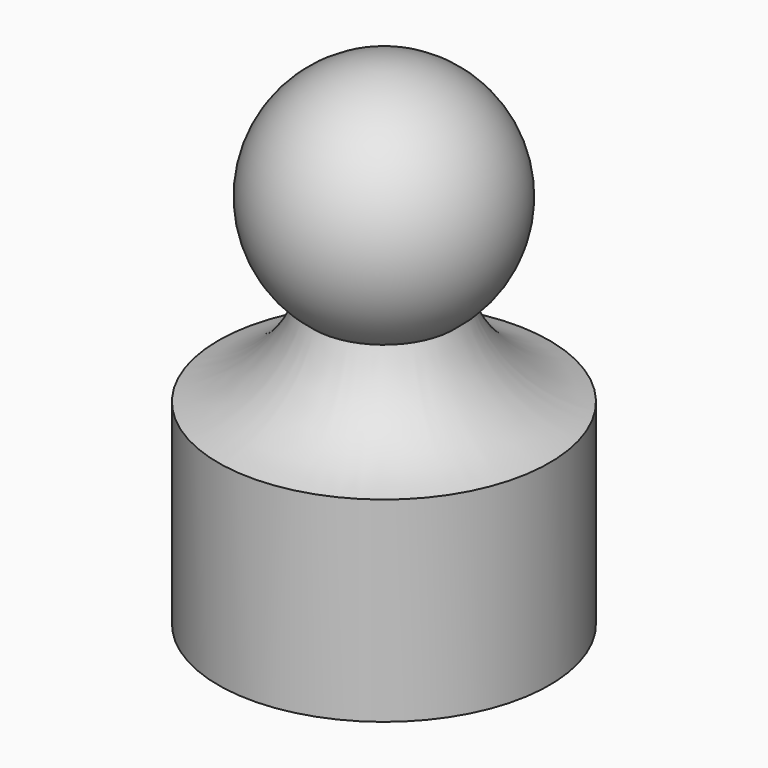
from build123d import *


# Not quite as in the source:
# - a fillet or chamfer that OpenCascade refuses, or shapes differently, is made with other operations: its cross-section is extruded or revolved along the edge and cut away or added
# - a feature names something its author has since deleted; it is built from what else it names


with BuildPart() as f1:
    # F0 (on Front) → F1 (revolve)
    with BuildSketch(Plane.XZ):
        with BuildLine():
            Line((-11, 13), (-11, 0))
            Line((-11, 0), (-7.7, 0))
            Line((-7.7, 0), (-8.1, 7.9899937422))
            ThreePointArc((-8.1, 7.9899937422), (-5.7275649276, 13.7175586698), (0, 16.0899937422))
            Line((0, 16.0899937422), (0, 17.2))
            ThreePointArc((0, 17.2), (-2.4667280394, 17.6003207651), (-4.680255449, 18.7601915949))
            ThreePointArc((-4.680255449, 18.7601915949), (-7.0630577198, 15.0275401408), (-11, 13))
        make_face()
        with BuildLine():
            ThreePointArc((0, 32.8), (-7.3996792349, 27.4667280394), (-4.680255449, 18.7601915949))
            ThreePointArc((-4.680255449, 18.7601915949), (-2.4667280394, 17.6003207651), (0, 17.2))
            Line((0, 17.2), (0, 32.8))
        make_face()
    revolve(axis=Axis((0, 0, 29.5921396464), (0, 0, 1)))

    # F2: chamfer of 2 x 1 on 1 edges, made by hand

    # F2_s1 → F2_t2 (revolve, cut)
    with BuildSketch(Plane.XZ):
        Polygon((-8.7, 0), (-7.8, 1.9974984355), (-7.7, 0), align=None)
    revolve(axis=Axis((0, 0, 0), (0, 0, 1)), mode=Mode.SUBTRACT)


solid = f1.part
